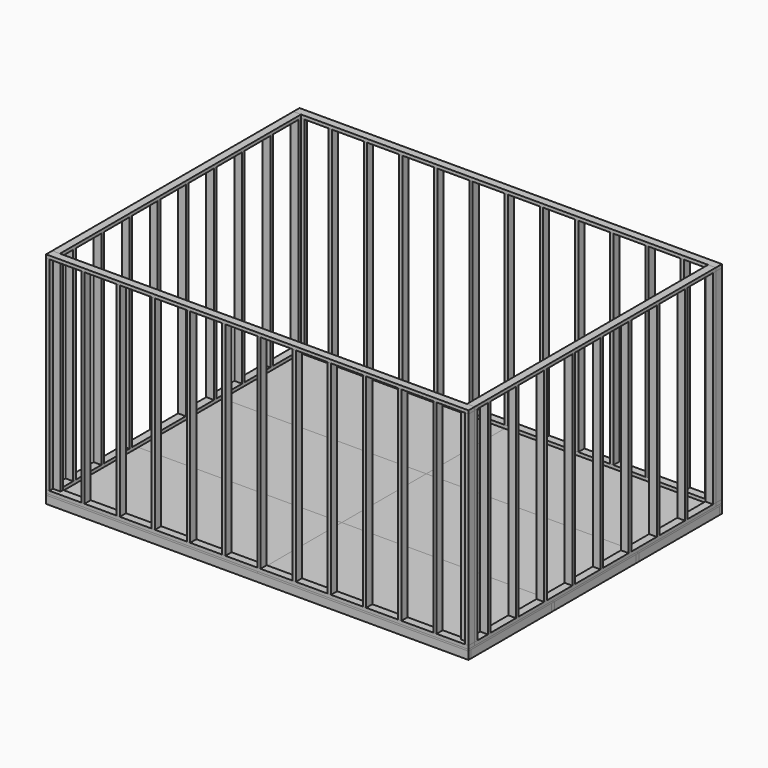
from build123d import *

# Parameters (mm, degrees)
F0_W      = 2438.4
F0_H      = 1219.2
F1_DEPTH  = 19.05
F7_W      = 4876.8
F7_H      = 88.9
F8_DEPTH  = 38.1
F9_W      = 4876.8
F9_H      = 38.1
F10_DEPTH = 88.9
F14_W     = 38.1
F14_H     = 1162.05
F15_DEPTH = 88.9
F29_DEPTH = 19.05
F33_W     = 88.9
F33_H     = 3479.8
F34_DEPTH = 38.1
F36_W     = 38.1
F36_H     = 88.9
F37_DEPTH = 2352.675
F65_W     = 88.9
F65_H     = 38.1
F66_DEPTH = 2352.675


with BuildPart() as f1:
    # F0 (on Top) → F1 (new body)
    with BuildSketch(Plane.XY):
        with Locations((1219.2, 609.6)):
            Rectangle(F0_W, F0_H)
    extrude(amount=-F1_DEPTH)


with BuildPart() as f2_1:
    # F2: copy of F1
    add(f1.part.moved(Location((2438.4, 0, 0))))


with BuildPart() as f3_1:
    # F3: copy of F1
    add(f1.part.moved(Location((0, 1219.2, 0))))


with BuildPart() as f4_1:
    # F4: copy of F3_1
    add(f3_1.part.moved(Location((2438.4, 0, 0))))


with BuildPart() as f5_1:
    # F5: copy of F3_1
    add(f3_1.part.moved(Location((0, 1219.2, 0))))


with BuildPart() as f6_1:
    # F6: copy of F4_1
    add(f4_1.part.moved(Location((0, 1219.2, 0))))


with BuildPart() as f8:
    # F7 (on Top) → F8 (new body)
    with BuildSketch(Plane.XY):
        with Locations((2438.4, 44.45)):
            Rectangle(F7_W, F7_H)
    extrude(amount=F8_DEPTH)


with BuildPart() as f10:
    # F9 (on face) → F10 (new body)
    with BuildSketch(Plane(origin=(0, 0, -19.05), x_dir=(1, 0, 0), z_dir=(0, 0, -1))):
        with Locations((2438.4, -19.05)):
            Rectangle(F9_W, F9_H)
    extrude(amount=F10_DEPTH)


with BuildPart() as f11_1:
    # F11: copy of F10
    add(f10.part.moved(Location((0, 1200.15, 0))))


with BuildPart() as f12_1:
    # F12: copy of F11_1
    add(f11_1.part.moved(Location((0, 1219.2, 0))))


with BuildPart() as f13_1:
    # F13: copy of F12_1
    add(f12_1.part.moved(Location((0, 1200.15, 0))))


with BuildPart() as f15:
    # F14 (on face) → F15 (new body)
    with BuildSketch(Plane(origin=(0, 0, -19.05), x_dir=(1, 0, 0), z_dir=(0, 0, -1))):
        with Locations((4857.75, -3036.8522449493)):
            Rectangle(F14_W, F14_H)
    extrude(amount=F15_DEPTH)


with BuildPart() as f15_1:
    # F16: moved
    add(f15.part.moved(Location((0, 1.6227550507, 0))))


with BuildPart() as f17_1:
    # F17: copy of F15
    add(f15_1.part.moved(Location((-2438.4, 0, 0))))


with BuildPart() as f17_1_1:
    # F18: moved
    add(f17_1.part.moved(Location((19.05, 0, 0))))


with BuildPart() as f19_1:
    # F19: copy of F17_1
    add(f17_1_1.part.moved(Location((-2419.35, 0, 0))))


with BuildPart() as f20_1:
    # F20: copy of F15
    add(f15_1.part.moved(Location((0, -1257.3, 0))))


with BuildPart() as f20_1_1:
    # F21: moved
    add(f20_1.part.moved(Location((0, 38.1, 0))))


with BuildPart() as f23_1:
    # F23: copy of F19_1
    add(f19_1.part.moved(Location((0, -2400.3, 0))))


with BuildPart() as f23_1_1:
    # F24: moved
    add(f23_1.part.moved(Location((0, -19.05, 0))))


with BuildPart() as f25_1:
    # F25: copy of F17_1
    add(f17_1_1.part.moved(Location((0, -2419.35, 0))))


with BuildPart() as f26_1:
    # F26: copy of F15
    add(f15_1.part.moved(Location((0, -2419.35, 0))))


with BuildPart() as f28_1:
    # F28: copy of F15
    add(f15_1.part.moved(Location((0, -1219.2, 0))))

    # F29 (add): a face of the model
    f29_faces = [f28_1.faces().sort_by_distance(p)[0] for p in [
        (4857.75, 2400.3, -63.5),
    ]]
    extrude(f29_faces, amount=F29_DEPTH)


with BuildPart() as f30_1:
    # F30: copy of F28_1
    add(f28_1.part.moved(Location((-2419.35, 0, 0))))


with BuildPart() as f31_1:
    # F31: copy of F30_1
    add(f30_1.part.moved(Location((-2419.35, 0, 0))))


with BuildPart() as f32_1:
    # F32: copy of F8
    add(f8.part.moved(Location((0, 3568.7, 0))))


with BuildPart() as f34:
    # F33 (on face) → F34 (new body)
    with BuildSketch(Plane.XY.offset(38.1)):
        with Locations((44.45, 1828.8)):
            Rectangle(F33_W, F33_H)
    extrude(amount=-F34_DEPTH)


with BuildPart() as f35_1:
    # F35: copy of F34
    add(f34.part.moved(Location((4787.9, 0, 0))))


with BuildPart() as f37:
    # F36 (on face) → F37 (new body)
    with BuildSketch(Plane.XY.offset(38.1)):
        with Locations((19.05, 3613.15)):
            Rectangle(F36_W, F36_H)
    extrude(amount=F37_DEPTH)


with BuildPart() as f38_1:
    # F38: copy of F37
    add(f37.part.moved(Location((406.4, 0, 0))))


with BuildPart() as f39_1:
    # F39: copy of F38_1
    add(f38_1.part.moved(Location((406.4, 0, 0))))


with BuildPart() as f40_1:
    # F40: copy of F39_1
    add(f39_1.part.moved(Location((406.4, 0, 0))))


with BuildPart() as f41_1:
    # F41: copy of F40_1
    add(f40_1.part.moved(Location((406.4, 0, 0))))


with BuildPart() as f42_1:
    # F42: copy of F41_1
    add(f41_1.part.moved(Location((406.4, 0, 0))))


with BuildPart() as f43_1:
    # F43: copy of F42_1
    add(f42_1.part.moved(Location((406.4, 0, 0))))


with BuildPart() as f44_1:
    # F44: copy of F43_1
    add(f43_1.part.moved(Location((406.4, 0, 0))))


with BuildPart() as f45_1:
    # F45: copy of F44_1
    add(f44_1.part.moved(Location((406.4, 0, 0))))


with BuildPart() as f46_1:
    # F46: copy of F45_1
    add(f45_1.part.moved(Location((406.4, 0, 0))))


with BuildPart() as f47_1:
    # F47: copy of F46_1
    add(f46_1.part.moved(Location((406.4, 0, 0))))


with BuildPart() as f48_1:
    # F48: copy of F47_1
    add(f47_1.part.moved(Location((406.4, 0, 0))))


with BuildPart() as f49_1:
    # F49: copy of F48_1
    add(f48_1.part.moved(Location((368.3, 0, 0))))


with BuildPart() as f50_1:
    # F50: copy of F32_1
    add(f32_1.part.moved(Location((0, 0, 2390.775))))


with BuildPart() as f51_1:
    # F51: copy of F37
    add(f37.part.moved(Location((0, -3568.7, 0))))


with BuildPart() as f52_1:
    # F52: copy of F51_1
    add(f51_1.part.moved(Location((406.4, 0, 0))))


with BuildPart() as f53_1:
    # F53: copy of F52_1
    add(f52_1.part.moved(Location((406.4, 0, 0))))


with BuildPart() as f54_1:
    # F54: copy of F53_1
    add(f53_1.part.moved(Location((406.4, 0, 0))))


with BuildPart() as f55_1:
    # F55: copy of F54_1
    add(f54_1.part.moved(Location((406.4, 0, 0))))


with BuildPart() as f56_1:
    # F56: copy of F55_1
    add(f55_1.part.moved(Location((406.4, 0, 0))))


with BuildPart() as f57_1:
    # F57: copy of F56_1
    add(f56_1.part.moved(Location((406.4, 0, 0))))


with BuildPart() as f58_1:
    # F58: copy of F57_1
    add(f57_1.part.moved(Location((406.4, 0, 0))))


with BuildPart() as f59_1:
    # F59: copy of F58_1
    add(f58_1.part.moved(Location((406.4, 0, 0))))


with BuildPart() as f60_1:
    # F60: copy of F59_1
    add(f59_1.part.moved(Location((406.4, 0, 0))))


with BuildPart() as f61_1:
    # F61: copy of F60_1
    add(f60_1.part.moved(Location((406.4, 0, 0))))


with BuildPart() as f62_1:
    # F62: copy of F61_1
    add(f61_1.part.moved(Location((406.4, 0, 0))))


with BuildPart() as f63_1:
    # F63: copy of F49_1
    add(f49_1.part.moved(Location((0, -3568.7, 0))))


with BuildPart() as f64_1:
    # F64: copy of F50_1
    add(f50_1.part.moved(Location((0, -3568.7, 0))))


with BuildPart() as f66:
    # F65 (on face) → F66 (new body)
    with BuildSketch(Plane.XY.offset(38.1)):
        with Locations((44.45, 3549.65)):
            Rectangle(F65_W, F65_H)
    extrude(amount=F66_DEPTH)


with BuildPart() as f67_1:
    # F67: copy of F66
    add(f66.part.moved(Location((0, -406.4, 0))))


with BuildPart() as f68_1:
    # F68: copy of F67_1
    add(f67_1.part.moved(Location((0, -406.4, 0))))


with BuildPart() as f69_1:
    # F69: copy of F68_1
    add(f68_1.part.moved(Location((0, -406.4, 0))))


with BuildPart() as f70_1:
    # F70: copy of F69_1
    add(f69_1.part.moved(Location((0, -406.4, 0))))


with BuildPart() as f71_1:
    # F71: copy of F70_1
    add(f70_1.part.moved(Location((0, -406.4, 0))))


with BuildPart() as f72_1:
    # F72: copy of F71_1
    add(f71_1.part.moved(Location((0, -406.4, 0))))


with BuildPart() as f73_1:
    # F73: copy of F72_1
    add(f72_1.part.moved(Location((0, -406.4, 0))))


with BuildPart() as f74_1:
    # F74: copy of F73_1
    add(f73_1.part.moved(Location((0, -406.4, 0))))


with BuildPart() as f75_1:
    # F75: copy of F74_1
    add(f74_1.part)


with BuildPart() as f76_1:
    # F76: copy of F75_1
    add(f75_1.part.moved(Location((0, -190.5, 0))))


with BuildPart() as f77_1:
    # F77: copy of F34
    add(f34.part.moved(Location((0, 0, 2390.775))))


with BuildPart() as f78_1:
    # F78: copy of F76_1
    add(f76_1.part.moved(Location((4787.9, 0, 0))))


with BuildPart() as f79_1:
    # F79: copy of F75_1
    add(f75_1.part.moved(Location((4787.9, 0, 0))))


with BuildPart() as f80_1:
    # F80: copy of F73_1
    add(f73_1.part.moved(Location((4787.9, 0, 0))))


with BuildPart() as f81_1:
    # F81: copy of F72_1
    add(f72_1.part.moved(Location((4787.9, 0, 0))))


with BuildPart() as f82_1:
    # F82: copy of F71_1
    add(f71_1.part.moved(Location((4787.9, 0, 0))))


with BuildPart() as f83_1:
    # F83: copy of F70_1
    add(f70_1.part.moved(Location((4787.9, 0, 0))))


with BuildPart() as f83_2:
    # F83: copy of F69_1
    add(f69_1.part.moved(Location((4787.9, 0, 0))))


with BuildPart() as f84_1:
    # F84: copy of F68_1
    add(f68_1.part.moved(Location((4787.9, 0, 0))))


with BuildPart() as f85_1:
    # F85: copy of F67_1
    add(f67_1.part.moved(Location((4787.9, 0, 0))))


with BuildPart() as f86_1:
    # F86: copy of F77_1
    add(f77_1.part.moved(Location((4787.9, 0, 0))))


with BuildPart() as f87_1:
    # F87: copy of F78_1
    add(f78_1.part.moved(Location((-44.45, -38.1, 0))))


with BuildPart() as f87_1_1:
    # F88: moved
    add(f87_1.part.moved(Location((6.35, 0, 0))))


with BuildPart() as f63_1_1:
    # F88: moved
    add(f63_1.part.moved(Location((6.35, 0, 0))))


with BuildPart() as f87_1_2:
    # F89: moved
    add(f87_1_1.part.moved(Location((6.35, 0, 0))))


with BuildPart() as f90_1:
    # F90: copy of F76_1
    add(f76_1.part.moved(Location((38.1, -38.1, 0))))


with BuildPart() as f91_1:
    # F91: copy of F66
    add(f66.part.moved(Location((38.1, 38.1, 0))))


with BuildPart() as f92_1:
    # F92: copy of F66
    add(f66.part.moved(Location((4787.9, 0, 0))))


with BuildPart() as f93_1:
    # F93: copy of F92_1
    add(f92_1.part.moved(Location((-38.1, 38.1, 0))))


with BuildPart() as f63_1_2:
    # F94: moved
    add(f63_1_1.part.moved(Location((-6.35, 0, 0))))


with BuildPart() as f87_1_3:
    # F95: moved
    add(f87_1_2.part.moved(Location((-6.35, 0, 0))))


solid = Compound([f1.part, f2_1.part, f3_1.part, f4_1.part, f5_1.part, f6_1.part, f8.part, f10.part, f11_1.part, f12_1.part, f13_1.part, f15_1.part, f17_1_1.part, f19_1.part, f23_1_1.part, f25_1.part, f26_1.part, f28_1.part, f30_1.part, f31_1.part, f32_1.part, f34.part, f35_1.part, f37.part, f38_1.part, f39_1.part, f40_1.part, f41_1.part, f42_1.part, f43_1.part, f44_1.part, f45_1.part, f46_1.part, f47_1.part, f48_1.part, f49_1.part, f50_1.part, f51_1.part, f52_1.part, f53_1.part, f54_1.part, f55_1.part, f56_1.part, f57_1.part, f58_1.part, f59_1.part, f60_1.part, f61_1.part, f62_1.part, f64_1.part, f66.part, f67_1.part, f68_1.part, f69_1.part, f70_1.part, f71_1.part, f72_1.part, f73_1.part, f74_1.part, f75_1.part, f76_1.part, f77_1.part, f78_1.part, f79_1.part, f80_1.part, f81_1.part, f82_1.part, f83_1.part, f83_2.part, f84_1.part, f85_1.part, f86_1.part, f90_1.part, f91_1.part, f92_1.part, f93_1.part, f63_1_2.part, f87_1_3.part])
